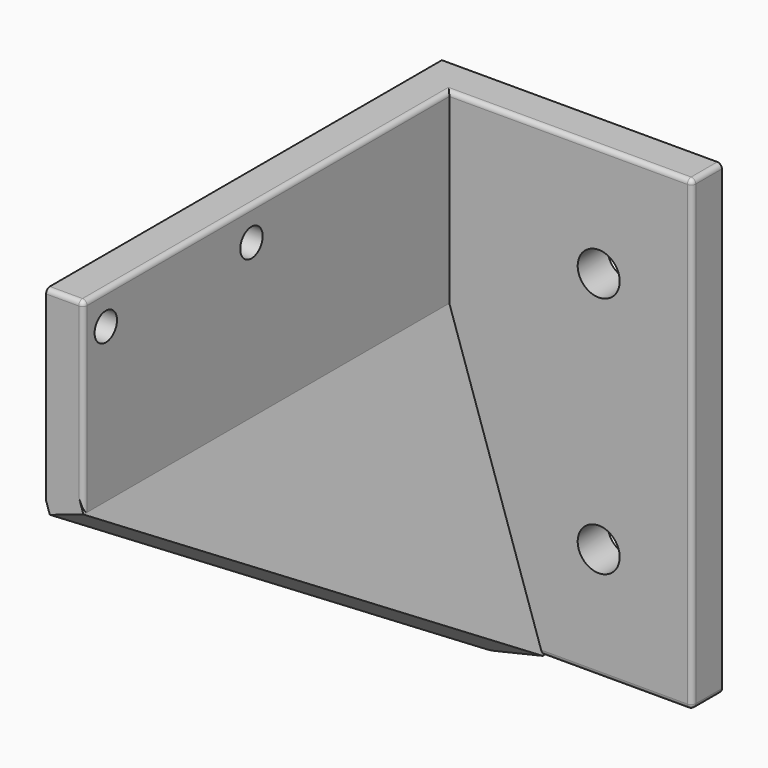
from build123d import *

# Parameters (mm, degrees)
F0_R         = 2.25
F0_W         = 4
F0_H         = 20
F1_DEPTH     = 4
F2_W         = 4
F2_H         = 20
F3_DEPTH     = 49
F5_DEPTH     = 13.2825661727
F6_T1_DEPTH  = 4.75
F6_T3_DEPTH  = 48.5
F6_T5_DEPTH  = 25.5
F6_T7_DEPTH  = 49
F6_T9_DEPTH  = 4.75
F6_T11_DEPTH = 7.7618980501
F6_S15_W     = 0.51
F6_S15_H     = 0.51
F6_T16_DEPTH = 0.51
F6_S21_W     = 0.51
F6_S21_H     = 0.51
F6_T22_DEPTH = 0.51
F6_S27_W     = 0.51
F6_S27_H     = 0.51
F6_T28_DEPTH = 0.51
F6_T34_DEPTH = 16.75
F6_T39_DEPTH = 20.75
F6_T45_DEPTH = 49.75
F6_T49_DEPTH = 26.75
F7_R         = 1.5
F8_DEPTH     = 30.001


# Not quite as in the source:
# - a fillet or chamfer that OpenCascade refuses, or shapes differently, is made with other operations: its cross-section is extruded or revolved along the edge and cut away or added


with BuildPart() as f1:
    # F0 (on Front) → F1 (new body)
    with BuildSketch(Plane.XZ):
        Polygon((15, 25), (-11, 25), (-11, 5), (-1, -25), (15, -25), align=None)
        with Locations((5, -13)):
            Circle(F0_R, mode=Mode.SUBTRACT)
        with Locations((5, 13)):
            Circle(F0_R, mode=Mode.SUBTRACT)
        with Locations((-13, 15)):
            Rectangle(F0_W, F0_H)
        Polygon((-11, 5), (-15, 5), (-5, -25), (-1, -25), align=None)
    extrude(amount=-F1_DEPTH)

    # F2 (on face) → F3 (join)
    with BuildSketch(Plane.XZ):
        with Locations((-13, 15)):
            Rectangle(F2_W, F2_H)
        Polygon((-11, 5), (-15, 5), (-5, -25), (-1, -25), align=None)
    extrude(amount=F3_DEPTH)

    # F4 (on face) → F5 (cut, through all)
    with BuildSketch(Plane(origin=(-8.4, 0, -2.8), x_dir=(0, 1, 0), z_dir=(0.9486832981, 0, 0.316227766))):
        Polygon((0, -23.4008546852), (-49, 8.2219219164), (-49, -23.4008546852), align=None)
    extrude(amount=-F5_DEPTH, mode=Mode.SUBTRACT)

    # F6: fillet of radius 0.5 on 9 edges, made by hand

    # F6_s2 → F6_t1 (cut)
    with BuildSketch(Plane.YZ.offset(-16.25)):
        with BuildLine():
            ThreePointArc((-48.5, 25), (-48.8535533906, 24.8535533906), (-49, 24.5))
            Line((-49, 24.5), (-49, 25))
            Line((-49, 25), (-48.5, 25))
        make_face()
    extrude(amount=F6_T1_DEPTH, mode=Mode.SUBTRACT)

    # F6_s4 → F6_t3 (cut)
    with BuildSketch(Plane.XZ):
        with BuildLine():
            ThreePointArc((-11.5, 25), (-11.1464466094, 24.8535533906), (-11, 24.5))
            Line((-11, 24.5), (-11, 25))
            Line((-11, 25), (-11.5, 25))
        make_face()
    extrude(amount=F6_T3_DEPTH, mode=Mode.SUBTRACT)

    # F6_s6 → F6_t5 (cut)
    with BuildSketch(Plane.YZ.offset(-11)):
        with BuildLine():
            ThreePointArc((0.5, 25), (0.1464466094, 24.8535533906), (0, 24.5))
            Line((0, 24.5), (0, 25))
            Line((0, 25), (0.5, 25))
        make_face()
    extrude(amount=F6_T5_DEPTH, mode=Mode.SUBTRACT)

    # F6_s8 → F6_t7 (cut)
    with BuildSketch(Plane.XY.offset(-24.5)):
        with BuildLine():
            ThreePointArc((15, 0.5), (14.8535533906, 0.1464466094), (14.5, 0))
            Line((14.5, 0), (15, 0))
            Line((15, 0), (15, 0.5))
        make_face()
    extrude(amount=F6_T7_DEPTH, mode=Mode.SUBTRACT)

    # F6_s10 → F6_t9 (cut)
    with BuildSketch(Plane.XZ.offset(-5.25)):
        with BuildLine():
            ThreePointArc((14.5, 25), (14.8535533906, 24.8535533906), (15, 24.5))
            Line((15, 24.5), (15, 25))
            Line((15, 25), (14.5, 25))
        make_face()
        with BuildLine():
            ThreePointArc((15, -24.5), (14.8535533906, -24.8535533906), (14.5, -25))
            Line((14.5, -25), (15, -25))
            Line((15, -25), (15, -24.5))
        make_face()
    extrude(amount=F6_T9_DEPTH, mode=Mode.SUBTRACT)

    # F6_s12 → F6_t11 (cut)
    with BuildSketch(Plane.XZ.offset(-4.9009490251)):
        with BuildLine():
            ThreePointArc((-4.63962039, -25), (-4.9319755323, -24.9056210926), (-5.113962039, -24.658113883))
            Line((-5.113962039, -24.658113883), (-5, -25))
            Line((-5, -25), (-4.63962039, -25))
        make_face()
    extrude(amount=F6_T11_DEPTH, mode=Mode.SUBTRACT)


with BuildPart() as f6_tool14:
    # F6_s15 → F6_t16 (new body)
    with BuildSketch(Plane.XY.offset(24.5)):
        with Locations((-11.245, -48.755)):
            Rectangle(F6_S15_W, F6_S15_H)
    extrude(amount=F6_T16_DEPTH)

    # F6_s17 → F6_t18 (revolve, cut)
    with BuildSketch(Plane(origin=(-11.5, -48.5, 24.5), x_dir=(-0.7071067812, 0.7071067812, 0), z_dir=(0.7071067812, 0.7071067812, 0))):
        with BuildLine():
            ThreePointArc((0, -0.5), (0.5, 0), (0, 0.5))
            Line((0, 0.5), (0, -0.5))
        make_face()
    revolve(axis=Axis((-11.5, -48.5, 24.5), (0, 0, 1)), mode=Mode.SUBTRACT)


with BuildPart() as f1_1:
    add(f1.part)

    # F6_t13: cut F6_tool14
    add(f6_tool14.part, mode=Mode.SUBTRACT)


with BuildPart() as f6_tool20:
    # F6_s21 → F6_t22 (new body)
    with BuildSketch(Plane.XY.offset(24.5)):
        with Locations((14.755, 0.245)):
            Rectangle(F6_S21_W, F6_S21_H)
    extrude(amount=F6_T22_DEPTH)

    # F6_s23 → F6_t24 (revolve, cut)
    with BuildSketch(Plane(origin=(14.5, 0.5, 24.5), x_dir=(-0.7071067812, 0.7071067812, 0), z_dir=(0.7071067812, 0.7071067812, 0))):
        with BuildLine():
            ThreePointArc((0, -0.5), (0.5, 0), (0, 0.5))
            Line((0, 0.5), (0, -0.5))
        make_face()
    revolve(axis=Axis((14.5, 0.5, 24.5), (0, 0, 1)), mode=Mode.SUBTRACT)


with BuildPart() as f1_2:
    add(f1_1.part)

    # F6_t19: cut F6_tool20
    add(f6_tool20.part, mode=Mode.SUBTRACT)


with BuildPart() as f6_tool26:
    # F6_s27 → F6_t28 (new body)
    with BuildSketch(Plane.YZ.offset(14.5)):
        with Locations((0.245, -24.755)):
            Rectangle(F6_S27_W, F6_S27_H)
    extrude(amount=F6_T28_DEPTH)

    # F6_s29 → F6_t30 (revolve, cut)
    with BuildSketch(Plane(origin=(14.5, 0.5, -24.5), x_dir=(0, 0.7071067812, 0.7071067812), z_dir=(0, 0.7071067812, -0.7071067812))):
        with BuildLine():
            ThreePointArc((0, -0.5), (0.5, 0), (0, 0.5))
            Line((0, 0.5), (0, -0.5))
        make_face()
    revolve(axis=Axis((14.5, 0.5, -24.5), (1, 0, 0)), mode=Mode.SUBTRACT)


with BuildPart() as f1_3:
    add(f1_2.part)

    # F6_t25: cut F6_tool26
    add(f6_tool26.part, mode=Mode.SUBTRACT)


with BuildPart() as f6_tool32:
    # F6_s33 → F6_t34 (new body)
    with BuildSketch(Plane.YZ.offset(-2.25)):
        with BuildLine():
            ThreePointArc((0, -24.5), (0.1464466094, -24.8535533906), (0.5, -25))
            Line((0.5, -25), (0, -25))
            Line((0, -25), (0, -24.5))
        make_face()
    extrude(amount=F6_T34_DEPTH)

    split(bisect_by=Plane(origin=(-8.4, 0, -2.8), x_dir=(0, 1, 0), z_dir=(0.9486832981, 0, 0.316227766)), keep=Keep.TOP)


with BuildPart() as f1_4:
    add(f1_3.part)

    # F6_t31: cut F6_tool32
    add(f6_tool32.part, mode=Mode.SUBTRACT)


with BuildPart() as f6_tool37:
    # F6_s38 → F6_t39 (new body)
    with BuildSketch(Plane.XY.offset(3.75)):
        with BuildLine():
            ThreePointArc((-11.5, -49), (-11.1464466094, -48.8535533906), (-11, -48.5))
            Line((-11, -48.5), (-11, -49))
            Line((-11, -49), (-11.5, -49))
        make_face()
    extrude(amount=F6_T39_DEPTH)

    split(bisect_by=Plane(origin=(-8.4, 0, -2.8), x_dir=(0, 1, 0), z_dir=(0.9486832981, 0, 0.316227766)), keep=Keep.TOP)


with BuildPart() as f1_5:
    add(f1_4.part)

    # F6_t36: cut F6_tool37
    add(f6_tool37.part, mode=Mode.SUBTRACT)


with BuildPart() as f6_tool43:
    # F6_s44 → F6_t45 (new body)
    with BuildSketch(Plane.XZ.offset(-1.25)):
        with BuildLine():
            ThreePointArc((-11.5, 25), (-11.1464466094, 24.8535533906), (-11, 24.5))
            Line((-11, 24.5), (-11, 25))
            Line((-11, 25), (-11.5, 25))
        make_face()
    extrude(amount=F6_T45_DEPTH)

    split(bisect_by=Plane.XZ, keep=Keep.BOTTOM)


with BuildPart() as f6_tool47:
    # F6_s48 → F6_t49 (new body)
    with BuildSketch(Plane.YZ.offset(14.5)):
        with BuildLine():
            ThreePointArc((0.5, 25), (0.1464466094, 24.8535533906), (0, 24.5))
            Line((0, 24.5), (0, 25))
            Line((0, 25), (0.5, 25))
        make_face()
    extrude(amount=-F6_T49_DEPTH)

    split(bisect_by=Plane.YZ.offset(-11), keep=Keep.BOTTOM)


with BuildPart() as f6_tool43_1:
    add(f6_tool43.part)

    # F6_t51: intersect F6_tool47
    add(f6_tool47.part, mode=Mode.INTERSECT)


with BuildPart() as f1_6:
    add(f1_5.part)

    # F6_t41: cut F6_tool43
    add(f6_tool43_1.part, mode=Mode.SUBTRACT)

    # F7 (on face) → F8 (cut, through all)
    with BuildSketch(Plane(origin=(-15, 0, 0), x_dir=(0, -1, 0), z_dir=(-1, 0, 0))):
        with Locations((26.5, 21.5)):
            Circle(F7_R)
        with Locations((46, 21.5)):
            Circle(F7_R)
    extrude(amount=-F8_DEPTH, mode=Mode.SUBTRACT)


solid = f1_6.part
